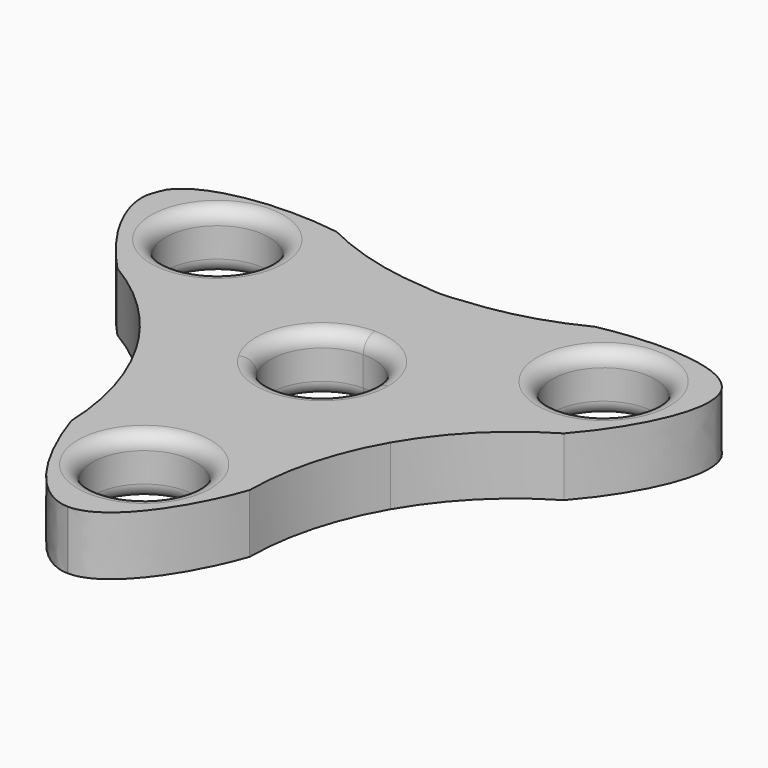
from build123d import *

# Parameters (mm, degrees)
F0_R     = 17.5
F1_DEPTH = 20
F2_R     = 5


# Not quite as in the source:
# - a feature names something its author has since deleted; it is built from what else it names


with BuildPart() as f1:
    # F0 (on Top) → F1 (new body)
    with BuildSketch(Plane.XY):
        with BuildLine():
            ThreePointArc((-0.8029759794, -107.3276413225), (-0.6770077139, -107.3305842091), (-0.551028741, -107.3330261089))
            add(Edge.make_bspline(
                [(-0.551028741, -107.3330261089), (11.8181523091, -107.461473966), (24.9052651001, -87.6452975434), (31.1277913127, -69.7459411731)],
                knots=[0.2489575342, 0.2489575342, 0.2489575342, 0.2489575342, 0.333331839, 0.333331839, 0.333331839, 0.333331839], degree=3))
            ThreePointArc((31.1277913127, -69.7459411731), (34.2703147589, -46.5679448448), (43.2491060822, -24.9698830388))
            Line((43.2491060822, -24.9698830388), (15.1554445662, -8.75))
            ThreePointArc((15.1554445662, -8.75), (0, -17.5), (-15.1554445662, -8.75))
            Line((-15.1554445662, -8.75), (-43.2831772417, -24.9895540319))
            ThreePointArc((-43.2831772417, -24.9895540319), (-34.3639851715, -45.8098967668), (-30.7884242712, -68.1762559483))
            add(Edge.make_bspline(
                [(-30.7884242712, -68.1762559483), (-24.9091046437, -86.1543987507), (-13.2460019559, -106.9245217626), (-0.8029759794, -107.3276413225)],
                knots=[0.1634370226, 0.1634370226, 0.1634370226, 0.1634370226, 0.2483844308, 0.2483844308, 0.2483844308, 0.2483844308], degree=3))
        make_face()
        with Locations((0, -75.6542630794)):
            Circle(F0_R, mode=Mode.SUBTRACT)
        with BuildLine():
            Line((15.1554445662, -8.75), (43.2491060822, -24.9698830388))
            ThreePointArc((43.2491060822, -24.9698830388), (57.4641806171, -6.3949907545), (75.9656525231, 7.9155125461))
            add(Edge.make_bspline(
                [(75.9656525231, 7.9155125461), (88.3019417057, 21.9444843566), (99.0200166091, 42.4631515807), (93.1968089359, 53.246587896)],
                knots=[0.4980383956, 0.4980383956, 0.4980383956, 0.4980383956, 0.5814448504, 0.5814448504, 0.5814448504, 0.5814448504], degree=3))
            ThreePointArc((93.1968089359, 53.246587896), (93.0778520452, 53.4582073651), (92.9572772103, 53.6689091704))
            add(Edge.make_bspline(
                [(92.9572772309, 53.6689091323), (86.5751209743, 64.3925439745), (62.811229058, 64.7841921161), (44.1380127183, 61.0160283089)],
                knots=[0.5825469337, 0.5825469337, 0.5825469337, 0.5825469337, 0.6675409578, 0.6675409578, 0.6675409578, 0.6675409578], degree=3))
            ThreePointArc((44.1380127381, 61.0160283086), (43.9116000862, 60.901053892), (43.6848880533, 60.7866709406))
            ThreePointArc((43.6848880533, 60.7866709406), (25.7919775423, 53.9031742146), (6.8965083627, 50.6628010548))
            add(Edge.make_bspline(
                [(6.8965083627, 50.6628010548), (4.5739652958, 50.280943855), (2.2831775194, 50.0716978343), (0, 50.097151764)],
                knots=[0.7347669892, 0.7347669892, 0.7347669892, 0.7347669892, 0.7491083365, 0.7491083365, 0.7491083365, 0.7491083365], degree=3))
            Line((0, 50.097151764), (0, 17.5))
            ThreePointArc((0, 17.5), (12.3743686708, 12.3743686708), (17.5, 0))
            ThreePointArc((17.5, 0), (16.9037019601, -4.5293332893), (15.1554445662, -8.75))
        make_face()
        with Locations((65.5185137313, 37.8271315397)):
            Circle(F0_R, mode=Mode.SUBTRACT)
        with BuildLine():
            add(Edge.make_bspline(
                [(-43.6481574505, 60.7516855355), (-62.440250746, 63.7299483995), (-87.0795012181, 61.5392674073), (-94.1887599838, 51.3128513788)],
                knots=[0.8301910028, 0.8301910028, 0.8301910028, 0.8301910028, 0.9144937287, 0.9144937287, 0.9144937287, 0.9144937287], degree=3))
            ThreePointArc((-94.1887599838, 51.3128513788), (-95.3750569752, 48.4306444144), (-96.272426733, 45.4458253151))
            add(Edge.make_bspline(
                [(-96.272426733, 45.4458253151), (-97.2953532658, 34.6779957553), (-86.8668945977, 19.3887259528), (-75.9656525231, 7.9155125461)],
                knots=[0.928778392, 0.928778392, 0.928778392, 0.928778392, 1, 1, 1, 1], degree=3))
            ThreePointArc((-75.9656525231, 7.9155125461), (-64.1383408586, -0.3689777355), (-53.7881948507, -10.4383649091))
            ThreePointArc((-53.7881948507, -10.4383649091), (-48.1808952117, -17.4578234301), (-43.2831772417, -24.9895540319))
            Line((-43.2831772417, -24.9895540319), (-15.1554445662, -8.75))
            ThreePointArc((-15.1554445662, -8.75), (-15.1554445662, 8.75), (0, 17.5))
            Line((0, 17.5), (0, 50.097151764))
            add(Edge.make_bspline(
                [(0, 50.097151764), (-1.8145063432, 50.1173807285), (-3.6242060978, 50.2858446459), (-5.4447980162, 50.5684261256)],
                knots=[0.7491083365, 0.7491083365, 0.7491083365, 0.7491083365, 0.7605058146, 0.7605058146, 0.7605058146, 0.7605058146], degree=3))
            ThreePointArc((-5.4447980162, 50.5684261256), (-25.0693332151, 53.6985192443), (-43.6481574505, 60.7516855355))
        make_face()
        with Locations((-65.6861164256, 37.535338503)):
            Circle(F0_R, mode=Mode.SUBTRACT)
    extrude(amount=F1_DEPTH)

    # F2
    f2_edges = [f1.edges().sort_by_distance(p)[0] for p in [
        (-48.186116, 37.535339, 10),
        (-83.186116, 37.535339, 0),
        (-83.186116, 37.535339, 20),
        (-15.155445, -8.75, 10),
        (15.155445, 8.75, 0),
        (15.155445, 8.75, 20),
        (83.018514, 37.827132, 10),
        (48.018514, 37.827132, 0),
        (48.018514, 37.827132, 20),
        (17.5, -75.654263, 10),
        (-17.5, -75.654263, 0),
        (-17.5, -75.654263, 20),
    ]]
    fillet(f2_edges, radius=F2_R)


solid = f1.part
